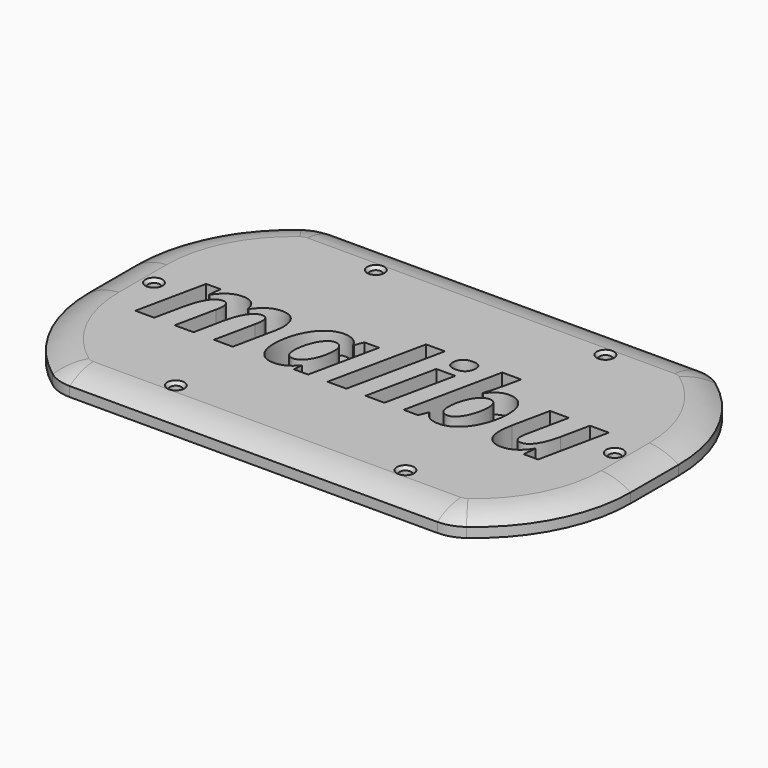
from build123d import *

# Parameters (mm, degrees)
F1_DEPTH       = 9.525
F2_R           = 12.7
F7_DEPTH       = 3.175
F9_D           = 3.7592
F9_CSINK_D     = 5.588
F9_CSINK_ANGLE = 82
F10_TEXT_SIZE  = 41.8302610648
F11_DEPTH      = 25.4
F13_DEPTH      = 3.175


# Not quite as in the source:
# - Text() gives the source's letters only with a copy of the font that has no kerning and outlines rounded to 1/6400 em; it was checked with that copy


with BuildPart() as f1:
    # F0 (on Top) → F1 (new body)
    with BuildSketch(Plane.XY):
        with BuildLine():
            Line((63.8113022832, 53.213), (-63.8113022832, 53.213))
            ThreePointArc((-63.8113022832, 53.213), (-81.731421563, 34.7013578741), (-88.265, 9.779))
            Line((-88.265, 9.779), (-88.265, -9.779))
            ThreePointArc((-88.265, -9.779), (-81.731421563, -34.7013578741), (-63.8113022832, -53.213))
            Line((-63.8113022832, -53.213), (63.8113022832, -53.213))
            ThreePointArc((63.8113022832, -53.213), (81.731421563, -34.7013578741), (88.265, -9.779))
            Line((88.265, -9.779), (88.265, 9.779))
            ThreePointArc((88.265, 9.779), (81.731421563, 34.7013578741), (63.8113022832, 53.213))
        make_face()
    extrude(amount=F1_DEPTH)

    # F2
    f2_edges = [f1.edges().sort_by_distance(p)[0] for p in [
        (63.811302, 53.213, 4.7625),
        (-63.811302, 53.213, 4.7625),
        (63.811302, -53.213, 4.7625),
        (-63.811302, -53.213, 4.7625),
    ]]
    fillet(f2_edges, radius=F2_R)

    # F5: sweep along a path in F3
    with BuildLine(Plane.XY.offset(9.525)) as f5_path:
        ThreePointArc((-59.9823542851, 43.688), (-60.9695019015, 43.5306422226), (-61.8588004755, 43.0741666667))
        ThreePointArc((-61.8588004755, 43.0741666667), (-74.278582681, 28.4440945668), (-78.74, 9.779))
        Line((-78.74, 9.779), (-78.74, -9.779))
        ThreePointArc((-78.74, -9.779), (-74.278582681, -28.4440945668), (-61.8588004755, -43.0741666667))
        ThreePointArc((-61.8588004755, -43.0741666667), (-60.9695019015, -43.5306422226), (-59.9823542851, -43.688))
        Line((-59.9823542851, -43.688), (59.9823542851, -43.688))
        ThreePointArc((59.9823542851, -43.688), (60.9695019015, -43.5306422226), (61.8588004755, -43.0741666667))
        ThreePointArc((61.8588004755, -43.0741666667), (74.278582681, -28.4440945668), (78.74, -9.779))
        Line((78.74, -9.779), (78.74, 9.779))
        ThreePointArc((78.74, 9.779), (74.278582681, 28.4440945668), (61.8588004755, 43.0741666667))
        ThreePointArc((61.8588004755, 43.0741666667), (60.9695019015, 43.5306422226), (59.9823542851, 43.688))
        Line((59.9823542851, 43.688), (-59.9823542851, 43.688))
    # F4 (on Front) → F5 (sweep, cut)
    with BuildSketch(Plane.XZ):
        with BuildLine():
            ThreePointArc((78.74, 9.525), (83.715434786, 8.576304358), (88.265, 6.35))
            Line((88.265, 6.35), (88.265, 10.795))
            Line((88.265, 10.795), (78.74, 10.795))
            Line((78.74, 10.795), (78.74, 9.525))
        make_face()
    sweep(path=f5_path.line, mode=Mode.SUBTRACT)

    # F6 (on face) → F7 (cut)
    with BuildSketch(Plane(origin=(0, 0, 0), x_dir=(1, 0, 0), z_dir=(0, 0, -1))):
        with BuildLine():
            ThreePointArc((59.9823542851, -53.213), (63.9309447509, -52.5835688902), (67.4881390468, -50.7576666667))
            ThreePointArc((67.4881390468, -50.7576666667), (82.7740248382, -32.7514240822), (88.265, -9.779))
            Line((88.265, -9.779), (88.265, 9.779))
            ThreePointArc((88.265, 9.779), (82.7740248382, 32.7514240822), (67.4881390468, 50.7576666667))
            ThreePointArc((67.4881390468, 50.7576666667), (63.9309447509, 52.5835688902), (59.9823542851, 53.213))
            Line((59.9823542851, 53.213), (-59.9823542851, 53.213))
            ThreePointArc((-59.9823542851, 53.213), (-63.9309447509, 52.5835688902), (-67.4881390468, 50.7576666667))
            ThreePointArc((-67.4881390468, 50.7576666667), (-82.7740248382, 32.7514240822), (-88.265, 9.779))
            Line((-88.265, 9.779), (-88.265, -9.779))
            ThreePointArc((-88.265, -9.779), (-82.7740248382, -32.7514240822), (-67.4881390468, -50.7576666667))
            ThreePointArc((-67.4881390468, -50.7576666667), (-63.9309447509, -52.5835688902), (-59.9823542851, -53.213))
            Line((-59.9823542851, -53.213), (59.9823542851, -53.213))
        make_face()
        with BuildLine():
            ThreePointArc((-59.8972810679, 33.1568312861), (-57.8701431096, 34.4663974856), (-55.5007685789, 34.925))
            Line((-55.5007685789, 34.925), (55.5007685789, 34.925))
            ThreePointArc((55.5007685789, 34.925), (57.8701431096, 34.4663974856), (59.8972810679, 33.1568312861))
            ThreePointArc((59.8972810679, 33.1568312861), (67.0750476967, 22.9310076394), (69.85, 10.749569188))
            Line((69.85, 10.749569188), (69.85, -8.808430812))
            ThreePointArc((69.85, -8.808430812), (67.4557440276, -22.0380987523), (59.8972810679, -33.1568312861))
            ThreePointArc((59.8972810679, -33.1568312861), (57.8701431096, -34.4663974856), (55.5007685789, -34.925))
            Line((55.5007685789, -34.925), (-55.5007685789, -34.925))
            ThreePointArc((-55.5007685789, -34.925), (-57.8701431096, -34.4663974856), (-59.8972810679, -33.1568312861))
            ThreePointArc((-59.8972810679, -33.1568312861), (-67.0750476967, -22.9310076394), (-69.85, -10.749569188))
            Line((-69.85, -10.749569188), (-69.85, 10.749569188))
            ThreePointArc((-69.85, 10.749569188), (-67.0750476967, 22.9310076394), (-59.8972810679, 33.1568312861))
        make_face(mode=Mode.SUBTRACT)
    extrude(amount=-F7_DEPTH, mode=Mode.SUBTRACT)

    # F9 (through all)
    with Locations(Plane.XY.offset(9.525)):
        with Locations((-75.0565700863, 0), (-35.2991081384, 40.7924), (39.6308918616, 40.7924), (75.3114299137, 0), (39.6308918616, -40.7924), (-35.2991081384, -40.7924)):
            CounterSinkHole(F9_D / 2, F9_CSINK_D / 2, counter_sink_angle=F9_CSINK_ANGLE)

    # F10 (on face) → F11 (cut)
    with BuildSketch(Plane.XY.offset(9.525)):
        with Locations((-69.85, -15.0555879667)):
            Text('malibu', F10_TEXT_SIZE, font='Open Sans', font_style=FontStyle.BOLDITALIC, text_align=(TextAlign.LEFT, TextAlign.BOTTOM))
    extrude(amount=-F11_DEPTH, mode=Mode.SUBTRACT)


with BuildPart() as f13:
    # F12 (on face) → F13 (new body)
    with BuildSketch(Plane(origin=(0, 0, 0), x_dir=(1, 0, 0), z_dir=(0, 0, -1))):
        Polygon((-19.0788796657, 16.6199764467), (-25.2896366783, 15.2974798189), (-20.2170954223, -8.5243738754), (-14.0063384097, -7.2018772477), align=None)
    extrude(amount=-F13_DEPTH)


with BuildPart() as f13b:
    # F12 (on face) → F13, piece 2 (new body)
    with BuildSketch(Plane(origin=(0, 0, 0), x_dir=(1, 0, 0), z_dir=(0, 0, -1))):
        Polygon((31.2478884091, 15.8846895497), (25.0359603176, 14.5677045893), (30.0877924895, -9.2606754809), (36.2997205811, -7.9436905205), align=None)
    extrude(amount=-F13_DEPTH)


solid = Compound([f1.part, f13.part, f13b.part])
